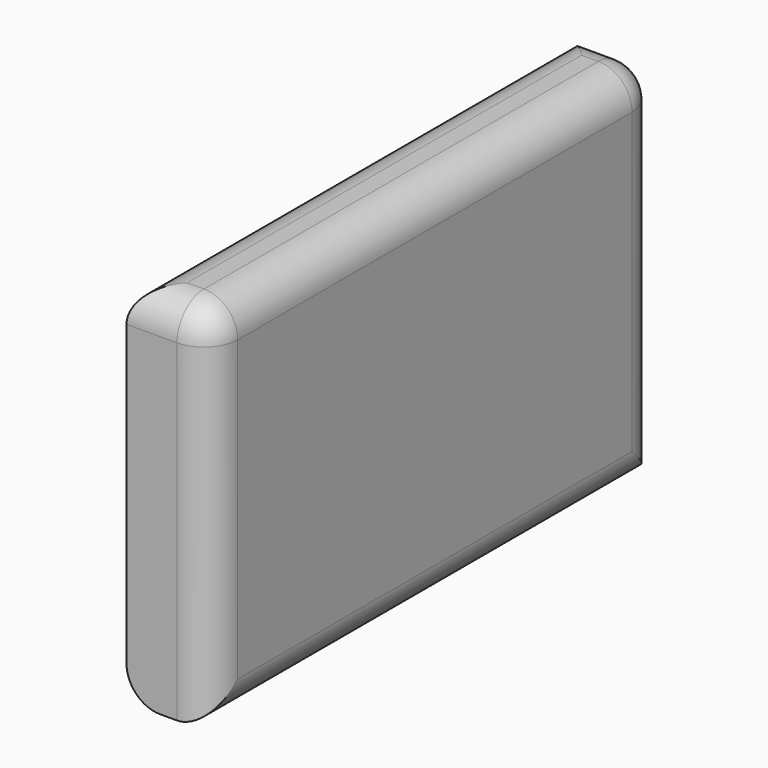
from build123d import *

# Parameters (mm, degrees)
F0_W         = 84.5384001732
F0_H         = 55.2411712706
F1_DEPTH     = 12.7
F2_R         = 5.08
F3_R         = 5.08
F4_T         = -2.54
F5_TEXT_SIZE = 58.4397691795
F6_DEPTH     = 12.7


# Not quite as in the source:
# - a shell that OpenCascade refuses in one call is made with other operations: the cavity is built on its own and cut out
# - Text() gives the source's letters only with a copy of the font that has no kerning and outlines rounded to 1/6400 em; it was checked with that copy


with BuildPart() as f1:
    # F0 (on Right) → F1 (new body)
    with BuildSketch(Plane.YZ):
        Rectangle(F0_W, F0_H)
    extrude(amount=F1_DEPTH)

    # F2
    f2_edges = [f1.edges().sort_by_distance(p)[0] for p in [
        (6.35, 42.2692, 27.620586),
        (6.35, -42.2692, 27.620586),
        (0, 0, 27.620586),
        (12.7, 0, 27.620586),
        (12.7, 42.2692, 0),
        (12.7, -42.2692, 0),
        (12.7, 0, -27.620586),
    ]]
    fillet(f2_edges, radius=F2_R)

    # F3
    f3_edges = [f1.edges().sort_by_distance(p)[0] for p in [
        (0, 0, -27.620586),
    ]]
    fillet(f3_edges, radius=F3_R)

    # F4: a shell. OpenCascade refuses it in one call, so the cavity is built on its own and cut out:
    # the body offset inwards by the wall thickness, plus a prism from it out through each open face.
    f4_core = offset(f1.part, amount=F4_T, mode=Mode.PRIVATE)
    f4_exits = [f4_core.faces().sort_by_distance(p)[0] for p in [
        (2.54, 0, 0),
    ]]
    add(f4_core, mode=Mode.SUBTRACT)
    extrude(f4_exits, amount=-F4_T, mode=Mode.SUBTRACT)

    # F5 (on face) → F6 (join)
    with BuildSketch(Plane(origin=(10.16, 0, 0), x_dir=(0, -1, 0), z_dir=(-1, 0, 0))):
        with Locations((-37.3671616869, -19.5360481739)):
            Text('RB', F5_TEXT_SIZE, font='Open Sans', text_align=(TextAlign.LEFT, TextAlign.BOTTOM))
    extrude(amount=F6_DEPTH)


solid = f1.part
